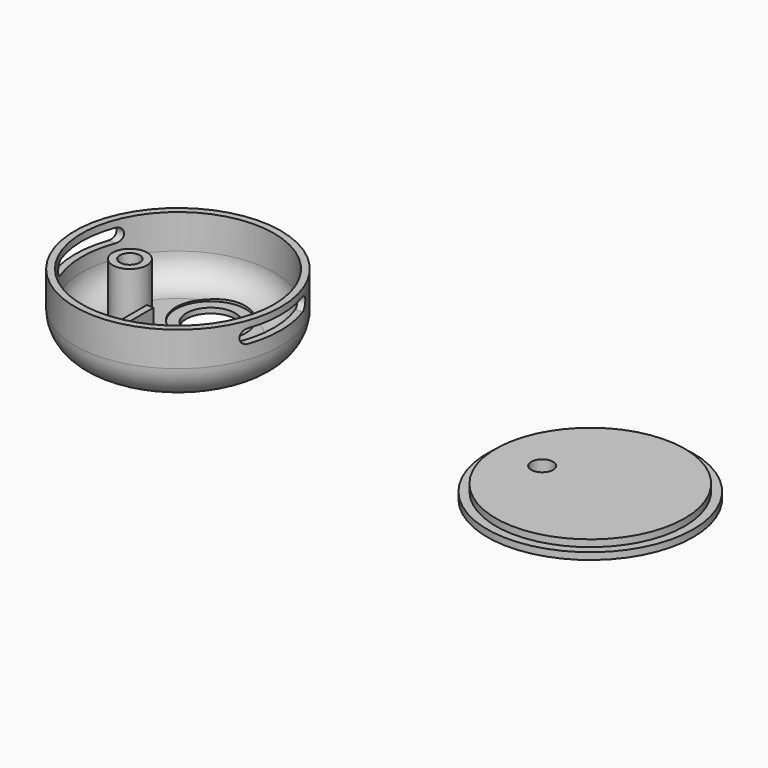
from build123d import *

# Parameters (mm, degrees)
F0_R      = 15
F1_DEPTH  = 10
F2_R      = 5
F3_T      = -1
F4_W      = 6.8
F4_H      = 7.7
F4_R      = 3.55
F5_DEPTH  = 1
F6_DEPTH  = 0.25
F7_DEPTH  = 3
F8_R      = 2.5
F8_R_2    = 1.45
F9_DEPTH  = 8
F12_REACH = 42.1665250606
F13_R     = 13.75
F14_DEPTH = 2
F13_R_2   = 15
F15_DEPTH = 1
F16_R     = 1.6
F17_DEPTH = 2


# Not quite as in the source:
# - a pattern or mirror of a feature is missing from the dataset's text; its kind, count and spacing are read off the source's solid


with BuildPart() as f1:
    # F0 (on Top) → F1 (new body)
    with BuildSketch(Plane.XY):
        Circle(F0_R)
    extrude(amount=F1_DEPTH)

    # F2
    f2_edges = [f1.edges().sort_by_distance(p)[0] for p in [
        (-15, 0, 0),
    ]]
    fillet(f2_edges, radius=F2_R)

    # F3
    f3_openings = [f1.faces().sort_by_distance(p)[0] for p in [
        (0, 0, 10),
    ]]
    offset(amount=F3_T, openings=f3_openings)

    # F4 (on face) → F5 (cut, through all)
    with BuildSketch(Plane.XY.offset(1)):
        with Locations((0, -5.0236860273)):
            Rectangle(F4_W, F4_H)
        with Locations((0, 5.9763139727)):
            Circle(F4_R)
    extrude(amount=-F5_DEPTH, mode=Mode.SUBTRACT)

    # F4 (on face) → F6 (cut, symmetric)
    with BuildSketch(Plane.XY.offset(1)):
        with BuildLine():
            ThreePointArc((-3.9694419174, 9.1784274723), (-1.6979172862, 1.1672520174), (5.1, 5.9763139727))
            ThreePointArc((5.1, 5.9763139727), (4.8090619552, 7.6742312589), (3.9694419174, 9.1784274723))
            ThreePointArc((3.9694419174, 9.1784274723), (0, 10), (-3.9694419174, 9.1784274723))
        make_face()
        with Locations((0, 5.9763139727)):
            Circle(F4_R, mode=Mode.SUBTRACT)
        with BuildLine():
            ThreePointArc((-3.9694419174, 9.1784274723), (0, 10), (3.9694419174, 9.1784274723))
            ThreePointArc((3.9694419174, 9.1784274723), (0, 11.0763139727), (-3.9694419174, 9.1784274723))
        make_face()
    extrude(amount=F6_DEPTH, both=True, mode=Mode.SUBTRACT)

    # F4 (on face) → F7 (join)
    with BuildSketch(Plane.XY.offset(1)):
        with BuildLine():
            Line((-4.4, -0.1736860273), (-4.4, -8.9799777283))
            ThreePointArc((-4.4, -8.9799777283), (-3.0253826694, -9.5313723935), (-1.5844002758, -9.8736860273))
            Line((-1.5844002758, -9.8736860273), (1.5844002758, -9.8736860273))
            ThreePointArc((1.5844002758, -9.8736860273), (3.0253826694, -9.5313723935), (4.4, -8.9799777283))
            Line((4.4, -8.9799777283), (4.4, -0.1736860273))
            Line((4.4, -0.1736860273), (3.4, -0.1736860273))
            Line((3.4, -0.1736860273), (3.4, -1.1736860273))
            Line((3.4, -1.1736860273), (3.4, -8.8736860273))
            Line((3.4, -8.8736860273), (-3.4, -8.8736860273))
            Line((-3.4, -8.8736860273), (-3.4, -1.1736860273))
            Line((-3.4, -1.1736860273), (-3.4, -0.1736860273))
            Line((-3.4, -0.1736860273), (-4.4, -0.1736860273))
        make_face()
        with BuildLine():
            ThreePointArc((-1.5844002758, -9.8736860273), (-3.0253826694, -9.5313723935), (-4.4, -8.9799777283))
            Line((-4.4, -8.9799777283), (-4.4, -9.8736860273))
            Line((-4.4, -9.8736860273), (-1.5844002758, -9.8736860273))
        make_face()
        with BuildLine():
            Line((4.4, -9.8736860273), (4.4, -8.9799777283))
            ThreePointArc((4.4, -8.9799777283), (3.0253826694, -9.5313723935), (1.5844002758, -9.8736860273))
            Line((1.5844002758, -9.8736860273), (4.4, -9.8736860273))
        make_face()
    extrude(amount=F7_DEPTH)

    # F8 (on face) → F9 (join)
    with BuildSketch(Plane.XY.offset(1)):
        with Locations((-7, 0)):
            Circle(F8_R)
        with Locations((-7, 0)):
            Circle(F8_R_2, mode=Mode.SUBTRACT)
    extrude(amount=F9_DEPTH)

    f12_end = f1.faces().sort_by_distance((-14, 0, 7.5))[0]
    # F11 (on offset) → F12 (cut, up to a face of the model that its end follows)
    with BuildSketch(Plane.YZ.offset(-15)):
        with BuildLine():
            Line((-5, 7), (5, 7))
            ThreePointArc((5, 7), (6, 8), (5, 9))
            Line((5, 9), (-5, 9))
            ThreePointArc((-5, 9), (-6, 8), (-5, 7))
        make_face()
    f12_long = extrude(amount=F12_REACH, mode=Mode.PRIVATE)
    f12 = split(f12_long, bisect_by=f12_end, keep=Keep.ALL, mode=Mode.PRIVATE).solids().sort_by_distance((-15, 0, 8))[0]
    add(f12, mode=Mode.SUBTRACT)

    # F12_copies: F12 across plane
    add(f12.mirror(Plane(origin=(0, 0, 0), x_dir=(0, 0, 1), z_dir=(1, 0, 0))), mode=Mode.SUBTRACT)


with BuildPart() as f14:
    # F13 (on Top) → F14 (new body)
    with BuildSketch(Plane.XY):
        with Locations((60.0599460304, 0)):
            Circle(F13_R)
    extrude(amount=F14_DEPTH)

    # F13 (on Top) → F15 (join)
    with BuildSketch(Plane.XY):
        with Locations((60.0599460304, 0)):
            Circle(F13_R_2)
        with Locations((60.0599460304, 0)):
            Circle(F13_R, mode=Mode.SUBTRACT)
    extrude(amount=F15_DEPTH)

    # F16 (on face) → F17 (cut, through all)
    with BuildSketch(Plane.XY.offset(2)):
        with Locations((53.0599460304, 0)):
            Circle(F16_R)
    extrude(amount=-F17_DEPTH, mode=Mode.SUBTRACT)


solid = Compound([f1.part, f14.part])
